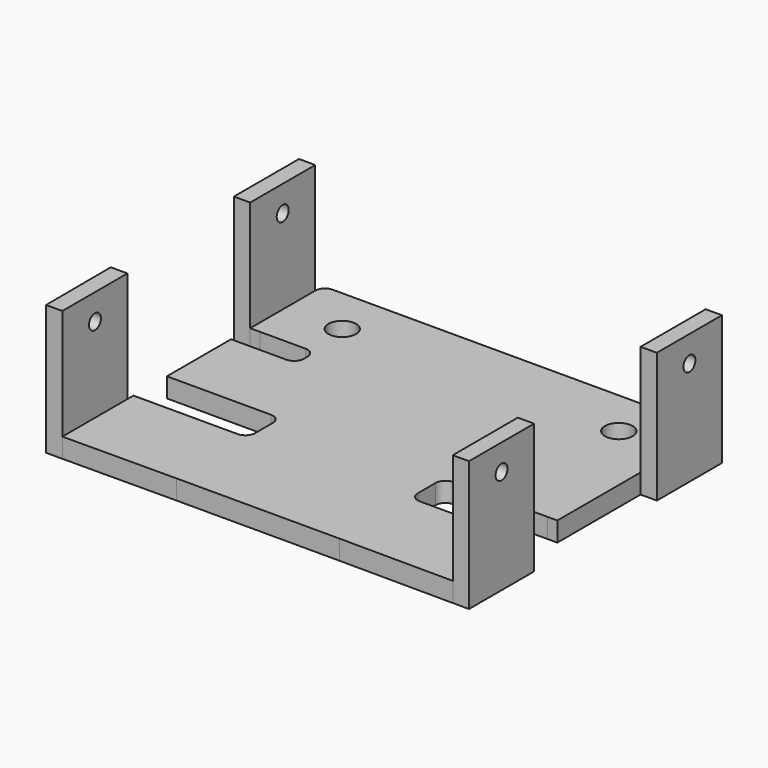
from build123d import *

# Parameters (mm, degrees)
F1_DEPTH  = 40
F0_R      = 4.2477627918
F2_DEPTH  = 6
F3_R      = 2.3
F4_DEPTH  = 5
F5_R      = 2.3
F6_DEPTH  = 6
F7_R      = 2.3
F8_DEPTH  = 6
F9_R      = 2.3
F10_DEPTH = 6


# Not quite as in the source:
# - ends of sketch curves that miss each other by under 0.0002 mm in the source are joined
# - a feature names something its author has since deleted; it is built from what else it names


with BuildPart() as f1:
    # F0 (on Top) → F1 (new body)
    with BuildSketch(Plane.XY):
        Polygon((64.9996812557, -4.4405678571), (59.9996996739, -4.4405506629), (59.999595637, -29.4405678569), (64.9995952845, -29.4405678569), align=None)
    extrude(amount=F1_DEPTH)

    # F7 (on face) → F8 (cut)
    with BuildSketch(Plane(origin=(64.9996965254, -0.0002235242, 0), x_dir=(3.4388e-06, 1, 0), z_dir=(1, -3.4388e-06, 0))):
        with Locations((-16.9403443329, 32)):
            Circle(F7_R)
    extrude(amount=-F8_DEPTH, mode=Mode.SUBTRACT)


with BuildPart() as f1b:
    # F0 (on Top) → F1, piece 2 (new body)
    with BuildSketch(Plane.XY):
        Polygon((65.0000812269, 67.727673769), (60, 67.727673769), (59.9998959633, 42.7276945771), (65.0000812269, 42.727673769), align=None)
    extrude(amount=F1_DEPTH)

    # F9 (on face) → F10 (cut)
    with BuildSketch(Plane.YZ.offset(65.0000812269)):
        with Locations((55.227673769, 32)):
            Circle(F9_R)
    extrude(amount=-F10_DEPTH, mode=Mode.SUBTRACT)


with BuildPart() as f1c:
    # F0 (on Top) → F1, piece 3 (new body)
    with BuildSketch(Plane.XY):
        Polygon((-59.9998959632, 42.7276737692), (-60, 67.727673769), (-65, 67.7276529616), (-64.9998959631, 42.7276529619), align=None)
    extrude(amount=F1_DEPTH)

    # F3 (on face) → F4 (cut)
    with BuildSketch(Plane(origin=(-64.9997181521, -0.0002704945, 0), x_dir=(4.1615e-06, -1, 0), z_dir=(-1, -4.1615e-06, 0))):
        with Locations((-55.2279234568, 32)):
            Circle(F3_R)
    extrude(amount=-F4_DEPTH, mode=Mode.SUBTRACT)


with BuildPart() as f1d:
    # F0 (on Top) → F1, piece 4 (new body)
    with BuildSketch(Plane.XY):
        Polygon((-59.999595637, -29.4405678569), (-59.9996996726, -4.4408566876), (-65.119768227, -4.4408566876), (-64.999595637, -29.4405678569), align=None)
    extrude(amount=F1_DEPTH)

    # F5 (on face) → F6 (cut)
    with BuildSketch(Plane(origin=(-65.139610072, -0.3131234436, 0), x_dir=(0.0048069036, -0.9999884468, 0), z_dir=(-0.9999884468, -0.0048069036, 0))):
        with Locations((16.6277809332, 32)):
            Circle(F5_R)
    extrude(amount=-F6_DEPTH, mode=Mode.SUBTRACT)


with BuildPart() as f2:
    # F0 (on Top) → F2 (new body)
    with BuildSketch(Plane.XY):
        with BuildLine():
            Line((57, 70.727673769), (0, 70.727673769))
            Line((0, 70.727673769), (-57, 70.727673769))
            ThreePointArc((-57, 70.727673769), (-59.1213203436, 69.8489941126), (-60, 67.727673769))
            Line((-60, 67.727673769), (-59.9998959632, 42.7276737692))
            Line((-59.9998959632, 42.7276737692), (-56.9999663575, 42.7276542423))
            Line((-56.9999663575, 42.7276542423), (-43, 42.727656483))
            Line((-43, 42.727656483), (59.9998959633, 42.7276729687))
            Line((59.9998959633, 42.7276729687), (60, 67.727673769))
            ThreePointArc((60, 67.727673769), (59.1213203436, 69.8489941126), (57, 70.727673769))
        make_face()
        with Locations((-42.5, 56.227673769)):
            Circle(F0_R, mode=Mode.SUBTRACT)
        with Locations((42.5, 56.227673769)):
            Circle(F0_R, mode=Mode.SUBTRACT)
        with BuildLine():
            Line((59.9997627961, 10.7276737687), (59.9998959633, 42.7276945771))
            Line((59.9998959633, 42.7276945771), (-43, 42.727656483))
            ThreePointArc((-43, 42.727656483), (-40.8786796564, 41.8489941126), (-40, 39.727673769))
            Line((-40, 39.727673769), (-40, 38.378118492))
            ThreePointArc((-40, 38.378118492), (-40.8786796564, 36.2567981484), (-43, 35.378118492))
            Line((-43, 35.378118492), (-56.9999512234, 35.378118492))
            Line((-56.9999512234, 35.378118492), (-59.9998653782, 35.3781060079))
            Line((-59.9998653782, 35.3781060079), (-59.9997627961, 10.727673769))
            Line((-59.9997627961, 10.727673769), (-57, 10.727673769))
            Line((-57, 10.727673769), (-27.9990918762, 10.727673769))
            ThreePointArc((-27.9990918762, 10.727673769), (-25.850534475, 9.8214027614), (-25.0000939277, 7.6501411647))
            Line((-25.0000939277, 7.6501411647), (-25.0000939277, 0.8731241727))
            ThreePointArc((-25.0000939277, 0.8731241727), (-25.8787735841, -1.2481961709), (-28.0000939277, -2.1268758273))
            Line((-28.0000939277, -2.1268758273), (-56.9996895647, -2.1268758273))
            Line((-56.9996895647, -2.1268758273), (-59.9996895647, -2.1268758273))
            Line((-59.9996895647, -2.1268758273), (-59.9996996726, -4.4408566876))
            Line((-59.9996996726, -4.4408566876), (-59.999595637, -29.4405678569))
            Line((-59.999595637, -29.4405678569), (-25, -29.272326231))
            Line((-25, -29.272326231), (0, -29.272326231))
            Line((0, -29.272326231), (25, -29.272326231))
            Line((25, -29.272326231), (59.999595637, -29.4405678569))
            Line((59.999595637, -29.4405678569), (59.9996996739, -4.4405506629))
            Line((59.9996996739, -4.4405506629), (59.9997093022, -2.1268758274))
            Line((59.9997093022, -2.1268758274), (56.9996895647, -2.1268655108))
            Line((56.9996895647, -2.1268655108), (27.9999896835, -2.1267657852))
            ThreePointArc((27.9999896835, -2.1267657852), (25.878676009, -1.2480824813), (25, 0.8732342148))
            Line((25, 0.8732342148), (25, 7.727673769))
            ThreePointArc((25, 7.727673769), (25.8786796564, 9.8489941126), (28, 10.727673769))
            Line((28, 10.727673769), (37, 10.727673769))
            Line((37, 10.727673769), (56.9996895647, 10.727673769))
            Line((56.9996895647, 10.727673769), (59.9997627961, 10.7276737687))
        make_face()
    extrude(amount=F2_DEPTH)


solid = Compound([f1.part, f1b.part, f1c.part, f1d.part, f2.part])
